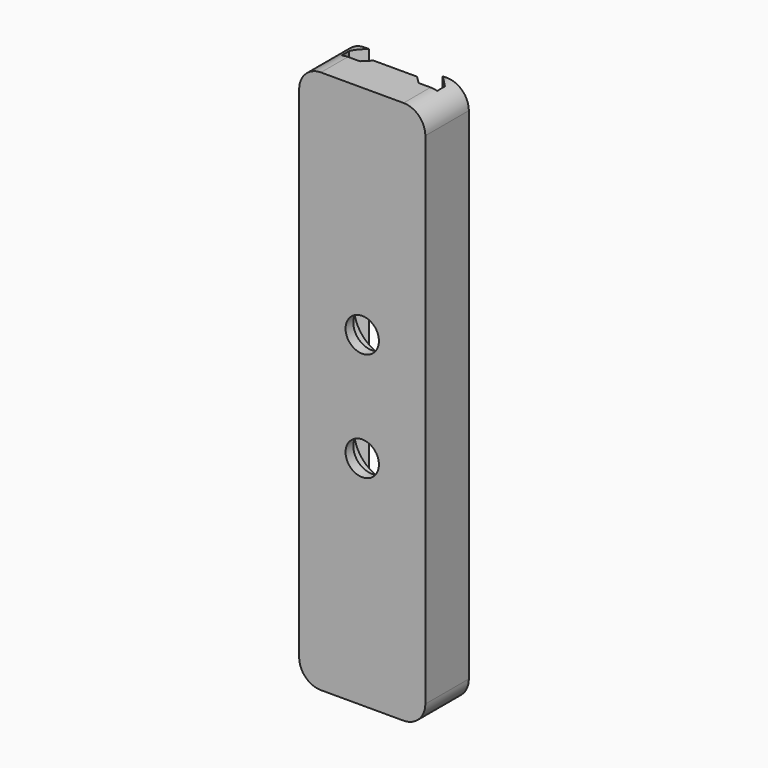
from build123d import *

# Parameters (mm, degrees)
F1_DEPTH       = 50
F3_D           = 3.4
F3_DEPTH       = 3
F3_CBORE_D     = 6.5
F3_CBORE_DEPTH = 2
F3_TIP         = 1.0214630523
F2_W           = 6
F2_H           = 1
F4_DEPTH       = 0.7
F5_T4_DEPTH    = 55.1433659759
F5_T9_DEPTH    = 55.1433659759
F5_T14_DEPTH   = 6.1433659759
F5_T19_DEPTH   = 6.1433659759
F5_T24_DEPTH   = 6.1433659759
F5_T29_DEPTH   = 6.1433659759
F6_T1_DEPTH    = 15


# Not quite as in the source:
# - a fillet or chamfer that OpenCascade refuses, or shapes differently, is made with other operations: its cross-section is extruded or revolved along the edge and cut away or added


with BuildPart() as f1:
    # F0 (on Top) → F1 (new body)
    with BuildSketch(Plane.XY):
        Polygon((-5.8, -2.5), (5.8, -2.5), (5.8, 2.5), (3.4, 2.5), (3.4, 1.5), (4.4, 1.5), (4.4, 0.6), (-4.4, 0.6), (-4.4, 1.5), (-3.4, 1.5), (-3.4, 2.5), (-5.8, 2.5), align=None)
    extrude(amount=F1_DEPTH)

    # F3
    with Locations(Plane(origin=(0, 0.6, 0), x_dir=(-1, 0, 0), z_dir=(0, 1, 0))):
        with Locations((0, 30), (0, 20)):
            CounterBoreHole(F3_D / 2, F3_CBORE_D / 2, F3_CBORE_DEPTH, depth=F3_DEPTH)
            with Locations((0, 0, -(F3_DEPTH + F3_TIP / 2))):  # 118° drill point
                Cone(0, F3_D / 2, F3_TIP, mode=Mode.SUBTRACT)

    # F2 (on face) → F4 (join)
    with BuildSketch(Plane(origin=(0, 0.6, 0), x_dir=(-1, 0, 0), z_dir=(0, 1, 0))):
        with Locations((0, 49.5)):
            Rectangle(F2_W, F2_H)
        with Locations((0, 0.5)):
            Rectangle(F2_W, F2_H)
    extrude(amount=F4_DEPTH)

    # F5: chamfer of 1 on 6 edges, made by hand


with BuildPart() as f5_tool2:
    # F5_s3 → F5_t4 (new body)
    with BuildSketch(Plane.XY.offset(-2.571682988)):
        Polygon((3.4, 2.5), (4.4, 1.5), (3.4, 1.5), align=None)
    extrude(amount=F5_T4_DEPTH)

    split(bisect_by=Plane.YZ.offset(4.4), keep=Keep.BOTTOM)


with BuildPart() as f1_1:
    add(f1.part)

    # F5_t1: cut F5_tool2
    add(f5_tool2.part, mode=Mode.SUBTRACT)


with BuildPart() as f5_tool7:
    # F5_s8 → F5_t9 (new body)
    with BuildSketch(Plane.XY.offset(-2.571682988)):
        Polygon((-4.4, 1.5), (-3.4, 2.5), (-3.4, 1.5), align=None)
    extrude(amount=F5_T9_DEPTH)

    split(bisect_by=Plane.YZ.offset(-4.4), keep=Keep.TOP)


with BuildPart() as f1_2:
    add(f1_1.part)

    # F5_t6: cut F5_tool7
    add(f5_tool7.part, mode=Mode.SUBTRACT)


with BuildPart() as f5_tool12:
    # F5_s13 → F5_t14 (new body)
    with BuildSketch(Plane.XY.offset(-2.571682988)):
        Polygon((-3, 0.3), (-2, 1.3), (-3, 1.3), align=None)
    extrude(amount=F5_T14_DEPTH)

    split(bisect_by=Plane.XZ.offset(-0.6), keep=Keep.BOTTOM)


with BuildPart() as f1_3:
    add(f1_2.part)

    # F5_t11: cut F5_tool12
    add(f5_tool12.part, mode=Mode.SUBTRACT)


with BuildPart() as f5_tool17:
    # F5_s18 → F5_t19 (new body)
    with BuildSketch(Plane.XY.offset(3.571682988)):
        Polygon((3, 0.3), (2, 1.3), (3, 1.3), align=None)
    extrude(amount=-F5_T19_DEPTH)

    split(bisect_by=Plane.XZ.offset(-0.6), keep=Keep.BOTTOM)


with BuildPart() as f1_4:
    add(f1_3.part)

    # F5_t16: cut F5_tool17
    add(f5_tool17.part, mode=Mode.SUBTRACT)


with BuildPart() as f5_tool22:
    # F5_s23 → F5_t24 (new body)
    with BuildSketch(Plane.XY.offset(52.571682988)):
        Polygon((3, 0.3), (2, 1.3), (3, 1.3), align=None)
    extrude(amount=-F5_T24_DEPTH)

    split(bisect_by=Plane.XZ.offset(-0.6), keep=Keep.BOTTOM)


with BuildPart() as f1_5:
    add(f1_4.part)

    # F5_t21: cut F5_tool22
    add(f5_tool22.part, mode=Mode.SUBTRACT)


with BuildPart() as f5_tool27:
    # F5_s28 → F5_t29 (new body)
    with BuildSketch(Plane.XY.offset(46.428317012)):
        Polygon((-3, 0.3), (-2, 1.3), (-3, 1.3), align=None)
    extrude(amount=F5_T29_DEPTH)

    split(bisect_by=Plane.XZ.offset(-0.6), keep=Keep.BOTTOM)


with BuildPart() as f1_6:
    add(f1_5.part)

    # F5_t26: cut F5_tool27
    add(f5_tool27.part, mode=Mode.SUBTRACT)

    # F6: fillet of radius 2 on 4 edges, made by hand

    # F6_s2 → F6_t1 (cut)
    with BuildSketch(Plane.XZ.offset(-7.5)):
        with BuildLine():
            ThreePointArc((5.8, 48), (5.2142135624, 49.4142135624), (3.8, 50))
            Line((3.8, 50), (5.8, 50))
            Line((5.8, 50), (5.8, 48))
        make_face()
        with BuildLine():
            ThreePointArc((-3.8, 50), (-5.2142135624, 49.4142135624), (-5.8, 48))
            Line((-5.8, 48), (-5.8, 50))
            Line((-5.8, 50), (-3.8, 50))
        make_face()
        with BuildLine():
            ThreePointArc((-3.8, 0), (-5.2142135624, 0.5857864376), (-5.8, 2))
            Line((-5.8, 2), (-5.8, 0))
            Line((-5.8, 0), (-3.8, 0))
        make_face()
        with BuildLine():
            ThreePointArc((5.8, 2), (5.2142135624, 0.5857864376), (3.8, 0))
            Line((3.8, 0), (5.8, 0))
            Line((5.8, 0), (5.8, 2))
        make_face()
    extrude(amount=F6_T1_DEPTH, mode=Mode.SUBTRACT)


solid = f1_6.part
